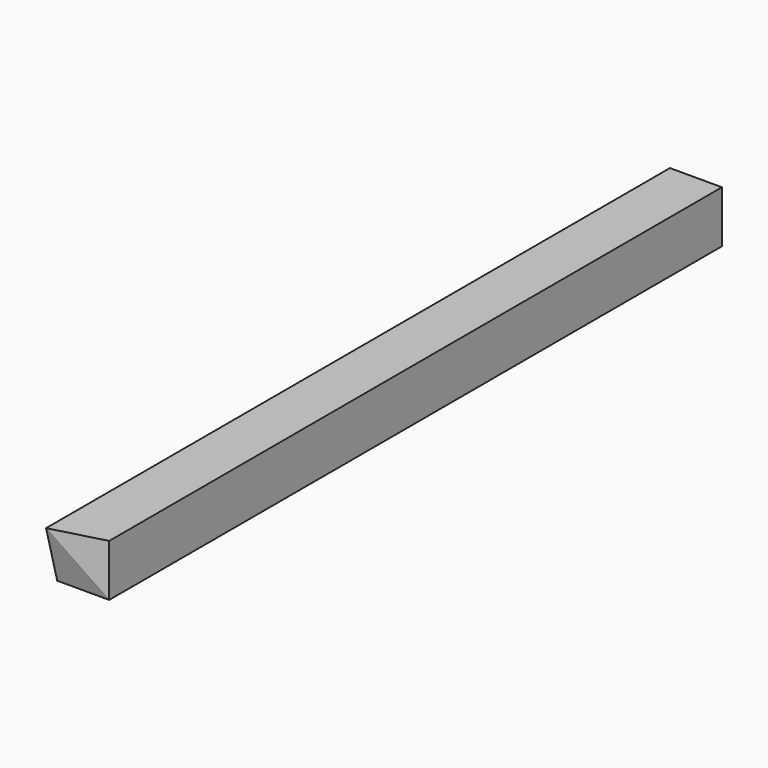
from build123d import *

# Parameters (mm, degrees)
F0_W     = 75
F0_H     = 75
F1_DEPTH = 1125
F2_SIZE2 = 20.096179
F2_SIZE  = 74.99999


# Not quite as in the source:
# - a fillet or chamfer is up to 0.001 mm smaller than in the source, because OpenCascade refuses the exact size


with BuildPart() as f1:
    # F0 (on Front) → F1 (new body)
    with BuildSketch(Plane.XZ):
        Rectangle(F0_W, F0_H)
    extrude(amount=F1_DEPTH)

    # F2 (size 75 and 20.0961894323 in the source; OpenCascade refuses exactly that, so slightly less here)
    f2_edges = [f1.edges().sort_by_distance(p)[0] for p in [
        (37.5, -1125, 0),
        (0, -1125, -37.5),
    ]]
    f2_side = f1.faces().sort_by_distance((0, -1125, 0))[0]
    chamfer(f2_edges, length=F2_SIZE, length2=F2_SIZE2, reference=f2_side)


solid = f1.part
